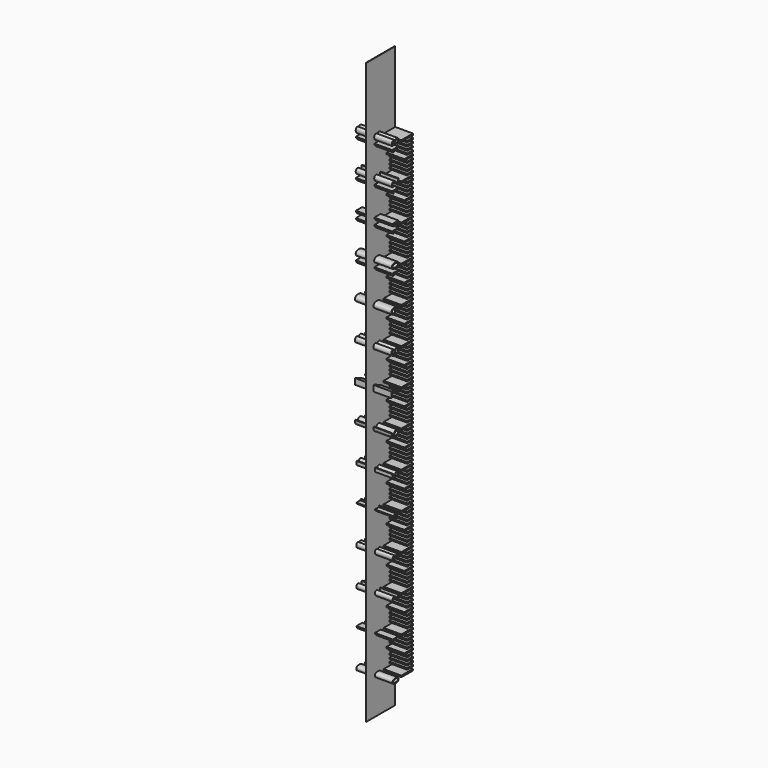
from build123d import *

# Parameters (mm, degrees)
F0_W           = 10
F0_H           = 160
F1_DEPTH       = 0.1
F2_W           = 4
F2_H           = 0.4
F2_W_2         = 3
F2_W_3         = 2
F2_TEXT_SIZE   = 2.7777777778
F2_TEXT_SIZE_2 = 3.4258994799
F2_TEXT_SIZE_3 = 3.0868508472
F3_DEPTH       = 5


# Not quite as in the source:
# - Text() gives the source's letters only with a copy of the font that has no kerning and outlines rounded to 1/6400 em; it was checked with that copy


with BuildPart() as f1:
    # F0 (on Right) → F1 (new body)
    with BuildSketch(Plane.YZ):
        with Locations((-15, 80)):
            Rectangle(F0_W, F0_H)
    extrude(amount=F1_DEPTH)

    # F2 (on Right) → F3 (join, symmetric)
    with BuildSketch(Plane.YZ):
        with Locations((-12, 10.2)):
            Rectangle(F2_W, F2_H)
        with Locations((-12, 20.2)):
            Rectangle(F2_W, F2_H)
        with Locations((-12, 30.2)):
            Rectangle(F2_W, F2_H)
        with Locations((-12, 40.2)):
            Rectangle(F2_W, F2_H)
        with Locations((-12, 50.2)):
            Rectangle(F2_W, F2_H)
        with Locations((-12, 60.2)):
            Rectangle(F2_W, F2_H)
        with Locations((-12, 70.2)):
            Rectangle(F2_W, F2_H)
        with Locations((-12, 80.2)):
            Rectangle(F2_W, F2_H)
        with Locations((-12, 90.2)):
            Rectangle(F2_W, F2_H)
        with Locations((-12, 100.2)):
            Rectangle(F2_W, F2_H)
        with Locations((-12, 110.2)):
            Rectangle(F2_W, F2_H)
        with Locations((-12, 120.2)):
            Rectangle(F2_W, F2_H)
        with Locations((-12, 130.2)):
            Rectangle(F2_W, F2_H)
        with Locations((-12, 140.2)):
            Rectangle(F2_W, F2_H)
        with Locations((-11.5, 15.2)):
            Rectangle(F2_W_2, F2_H)
        with Locations((-11, 11.2)):
            Rectangle(F2_W_3, F2_H)
        with Locations((-11, 12.2)):
            Rectangle(F2_W_3, F2_H)
        with Locations((-11, 13.2)):
            Rectangle(F2_W_3, F2_H)
        with Locations((-11, 14.2)):
            Rectangle(F2_W_3, F2_H)
        with Locations((-11, 16.2)):
            Rectangle(F2_W_3, F2_H)
        with Locations((-11, 17.2)):
            Rectangle(F2_W_3, F2_H)
        with Locations((-11, 18.2)):
            Rectangle(F2_W_3, F2_H)
        with Locations((-11, 19.2)):
            Rectangle(F2_W_3, F2_H)
        with Locations((-11, 22.2)):
            Rectangle(F2_W_3, F2_H)
        with Locations((-11, 21.2)):
            Rectangle(F2_W_3, F2_H)
        with Locations((-11, 23.2)):
            Rectangle(F2_W_3, F2_H)
        with Locations((-11, 28.2)):
            Rectangle(F2_W_3, F2_H)
        with Locations((-11.5, 25.2)):
            Rectangle(F2_W_2, F2_H)
        with Locations((-11, 29.2)):
            Rectangle(F2_W_3, F2_H)
        with Locations((-11, 24.2)):
            Rectangle(F2_W_3, F2_H)
        with Locations((-11, 26.2)):
            Rectangle(F2_W_3, F2_H)
        with Locations((-11, 27.2)):
            Rectangle(F2_W_3, F2_H)
        with Locations((-11, 32.2)):
            Rectangle(F2_W_3, F2_H)
        with Locations((-11, 31.2)):
            Rectangle(F2_W_3, F2_H)
        with Locations((-11, 33.2)):
            Rectangle(F2_W_3, F2_H)
        with Locations((-11, 38.2)):
            Rectangle(F2_W_3, F2_H)
        with Locations((-11.5, 35.2)):
            Rectangle(F2_W_2, F2_H)
        with Locations((-11, 39.2)):
            Rectangle(F2_W_3, F2_H)
        with Locations((-11, 34.2)):
            Rectangle(F2_W_3, F2_H)
        with Locations((-11, 36.2)):
            Rectangle(F2_W_3, F2_H)
        with Locations((-11, 37.2)):
            Rectangle(F2_W_3, F2_H)
        with Locations((-11, 42.2)):
            Rectangle(F2_W_3, F2_H)
        with Locations((-11, 41.2)):
            Rectangle(F2_W_3, F2_H)
        with Locations((-11, 43.2)):
            Rectangle(F2_W_3, F2_H)
        with Locations((-11, 48.2)):
            Rectangle(F2_W_3, F2_H)
        with Locations((-11.5, 45.2)):
            Rectangle(F2_W_2, F2_H)
        with Locations((-11, 49.2)):
            Rectangle(F2_W_3, F2_H)
        with Locations((-11, 44.2)):
            Rectangle(F2_W_3, F2_H)
        with Locations((-11, 46.2)):
            Rectangle(F2_W_3, F2_H)
        with Locations((-11, 47.2)):
            Rectangle(F2_W_3, F2_H)
        with Locations((-11, 52.2)):
            Rectangle(F2_W_3, F2_H)
        with Locations((-11, 51.2)):
            Rectangle(F2_W_3, F2_H)
        with Locations((-11, 53.2)):
            Rectangle(F2_W_3, F2_H)
        with Locations((-11, 58.2)):
            Rectangle(F2_W_3, F2_H)
        with Locations((-11.5, 55.2)):
            Rectangle(F2_W_2, F2_H)
        with Locations((-11, 59.2)):
            Rectangle(F2_W_3, F2_H)
        with Locations((-11, 54.2)):
            Rectangle(F2_W_3, F2_H)
        with Locations((-11, 56.2)):
            Rectangle(F2_W_3, F2_H)
        with Locations((-11, 57.2)):
            Rectangle(F2_W_3, F2_H)
        with Locations((-11, 62.2)):
            Rectangle(F2_W_3, F2_H)
        with Locations((-11, 61.2)):
            Rectangle(F2_W_3, F2_H)
        with Locations((-11, 63.2)):
            Rectangle(F2_W_3, F2_H)
        with Locations((-11, 68.2)):
            Rectangle(F2_W_3, F2_H)
        with Locations((-11.5, 65.2)):
            Rectangle(F2_W_2, F2_H)
        with Locations((-11, 69.2)):
            Rectangle(F2_W_3, F2_H)
        with Locations((-11, 64.2)):
            Rectangle(F2_W_3, F2_H)
        with Locations((-11, 66.2)):
            Rectangle(F2_W_3, F2_H)
        with Locations((-11, 67.2)):
            Rectangle(F2_W_3, F2_H)
        with Locations((-11, 72.2)):
            Rectangle(F2_W_3, F2_H)
        with Locations((-11, 71.2)):
            Rectangle(F2_W_3, F2_H)
        with Locations((-11, 73.2)):
            Rectangle(F2_W_3, F2_H)
        with Locations((-11, 78.2)):
            Rectangle(F2_W_3, F2_H)
        with Locations((-11.5, 75.2)):
            Rectangle(F2_W_2, F2_H)
        with Locations((-11, 79.2)):
            Rectangle(F2_W_3, F2_H)
        with Locations((-11, 74.2)):
            Rectangle(F2_W_3, F2_H)
        with Locations((-11, 76.2)):
            Rectangle(F2_W_3, F2_H)
        with Locations((-11, 77.2)):
            Rectangle(F2_W_3, F2_H)
        with Locations((-11, 82.2)):
            Rectangle(F2_W_3, F2_H)
        with Locations((-11, 81.2)):
            Rectangle(F2_W_3, F2_H)
        with Locations((-11, 83.2)):
            Rectangle(F2_W_3, F2_H)
        with Locations((-11, 88.2)):
            Rectangle(F2_W_3, F2_H)
        with Locations((-11.5, 85.2)):
            Rectangle(F2_W_2, F2_H)
        with Locations((-11, 89.2)):
            Rectangle(F2_W_3, F2_H)
        with Locations((-11, 84.2)):
            Rectangle(F2_W_3, F2_H)
        with Locations((-11, 86.2)):
            Rectangle(F2_W_3, F2_H)
        with Locations((-11, 87.2)):
            Rectangle(F2_W_3, F2_H)
        with Locations((-11, 92.2)):
            Rectangle(F2_W_3, F2_H)
        with Locations((-11, 91.2)):
            Rectangle(F2_W_3, F2_H)
        with Locations((-11, 93.2)):
            Rectangle(F2_W_3, F2_H)
        with Locations((-11, 98.2)):
            Rectangle(F2_W_3, F2_H)
        with Locations((-11.5, 95.2)):
            Rectangle(F2_W_2, F2_H)
        with Locations((-11, 99.2)):
            Rectangle(F2_W_3, F2_H)
        with Locations((-11, 94.2)):
            Rectangle(F2_W_3, F2_H)
        with Locations((-11, 96.2)):
            Rectangle(F2_W_3, F2_H)
        with Locations((-11, 97.2)):
            Rectangle(F2_W_3, F2_H)
        with Locations((-11, 102.2)):
            Rectangle(F2_W_3, F2_H)
        with Locations((-11, 101.2)):
            Rectangle(F2_W_3, F2_H)
        with Locations((-11, 103.2)):
            Rectangle(F2_W_3, F2_H)
        with Locations((-11, 108.2)):
            Rectangle(F2_W_3, F2_H)
        with Locations((-11.5, 105.2)):
            Rectangle(F2_W_2, F2_H)
        with Locations((-11, 109.2)):
            Rectangle(F2_W_3, F2_H)
        with Locations((-11, 104.2)):
            Rectangle(F2_W_3, F2_H)
        with Locations((-11, 106.2)):
            Rectangle(F2_W_3, F2_H)
        with Locations((-11, 107.2)):
            Rectangle(F2_W_3, F2_H)
        with Locations((-11, 112.2)):
            Rectangle(F2_W_3, F2_H)
        with Locations((-11, 111.2)):
            Rectangle(F2_W_3, F2_H)
        with Locations((-11, 113.2)):
            Rectangle(F2_W_3, F2_H)
        with Locations((-11, 118.2)):
            Rectangle(F2_W_3, F2_H)
        with Locations((-11.5, 115.2)):
            Rectangle(F2_W_2, F2_H)
        with Locations((-11, 119.2)):
            Rectangle(F2_W_3, F2_H)
        with Locations((-11, 114.2)):
            Rectangle(F2_W_3, F2_H)
        with Locations((-11, 116.2)):
            Rectangle(F2_W_3, F2_H)
        with Locations((-11, 117.2)):
            Rectangle(F2_W_3, F2_H)
        with Locations((-11, 122.2)):
            Rectangle(F2_W_3, F2_H)
        with Locations((-11, 121.2)):
            Rectangle(F2_W_3, F2_H)
        with Locations((-11, 123.2)):
            Rectangle(F2_W_3, F2_H)
        with Locations((-11, 128.2)):
            Rectangle(F2_W_3, F2_H)
        with Locations((-11.5, 125.2)):
            Rectangle(F2_W_2, F2_H)
        with Locations((-11, 129.2)):
            Rectangle(F2_W_3, F2_H)
        with Locations((-11, 124.2)):
            Rectangle(F2_W_3, F2_H)
        with Locations((-11, 126.2)):
            Rectangle(F2_W_3, F2_H)
        with Locations((-11, 127.2)):
            Rectangle(F2_W_3, F2_H)
        with Locations((-11, 132.2)):
            Rectangle(F2_W_3, F2_H)
        with Locations((-11, 131.2)):
            Rectangle(F2_W_3, F2_H)
        with Locations((-11, 133.2)):
            Rectangle(F2_W_3, F2_H)
        with Locations((-11, 138.2)):
            Rectangle(F2_W_3, F2_H)
        with Locations((-11.5, 135.2)):
            Rectangle(F2_W_2, F2_H)
        with Locations((-11, 139.2)):
            Rectangle(F2_W_3, F2_H)
        with Locations((-11, 134.2)):
            Rectangle(F2_W_3, F2_H)
        with Locations((-11, 136.2)):
            Rectangle(F2_W_3, F2_H)
        with Locations((-11, 137.2)):
            Rectangle(F2_W_3, F2_H)
        with Locations(Location((-17, 10.8151041667), (0, 0, -90))):
            Text('0', F2_TEXT_SIZE, font='Open Sans', text_align=(TextAlign.LEFT, TextAlign.BOTTOM))
        with Locations(Location((-15, 19.4251302083), (0, 0, 90))):
            Text('1', F2_TEXT_SIZE, font='Open Sans', text_align=(TextAlign.LEFT, TextAlign.BOTTOM))
        with Locations(Location((-15, 29.1903211806), (0, 0, 90))):
            Text('2', F2_TEXT_SIZE, font='Open Sans', text_align=(TextAlign.LEFT, TextAlign.BOTTOM))
        with Locations(Location((-15, 39.197265625), (0, 0, 90))):
            Text('3', F2_TEXT_SIZE, font='Open Sans', text_align=(TextAlign.LEFT, TextAlign.BOTTOM))
        with Locations(Location((-15, 49.1436631944), (0, 0, 90))):
            Text('4', F2_TEXT_SIZE, font='Open Sans', text_align=(TextAlign.LEFT, TextAlign.BOTTOM))
        with Locations(Location((-15, 59.1957465278), (0, 0, 90))):
            Text('5', F2_TEXT_SIZE, font='Open Sans', text_align=(TextAlign.LEFT, TextAlign.BOTTOM))
        with Locations(Location((-15, 68.993106731), (0, 0, 90))):
            Text('6', F2_TEXT_SIZE_2, font='Open Sans', text_align=(TextAlign.LEFT, TextAlign.BOTTOM))
        with Locations(Location((-15, 78.9965861602), (0, 0, 90))):
            Text('7', F2_TEXT_SIZE_2, font='Open Sans', text_align=(TextAlign.LEFT, TextAlign.BOTTOM))
        with Locations(Location((-15, 88.9981920505), (0, 0, 90))):
            Text('8', F2_TEXT_SIZE_2, font='Open Sans', text_align=(TextAlign.LEFT, TextAlign.BOTTOM))
        with Locations(Location((-15, 99.0014038313), (0, 0, 90))):
            Text('9', F2_TEXT_SIZE_2, font='Open Sans', text_align=(TextAlign.LEFT, TextAlign.BOTTOM))
        with Locations(Location((-15, 108.2117969506), (0, 0, 90))):
            Text('10', F2_TEXT_SIZE_3, font='Open Sans', text_align=(TextAlign.LEFT, TextAlign.BOTTOM))
        with Locations(Location((-15, 118.4787613169), (0, 0, 90))):
            Text('11', F2_TEXT_SIZE_3, font='Open Sans', text_align=(TextAlign.LEFT, TextAlign.BOTTOM))
        with Locations(Location((-15, 128.2178259562), (0, 0, 90))):
            Text('12', F2_TEXT_SIZE_3, font='Open Sans', text_align=(TextAlign.LEFT, TextAlign.BOTTOM))
        with Locations(Location((-15, 138.2255430833), (0, 0, 90))):
            Text('13', F2_TEXT_SIZE_3, font='Open Sans', text_align=(TextAlign.LEFT, TextAlign.BOTTOM))
    extrude(amount=F3_DEPTH, both=True)


solid = f1.part
